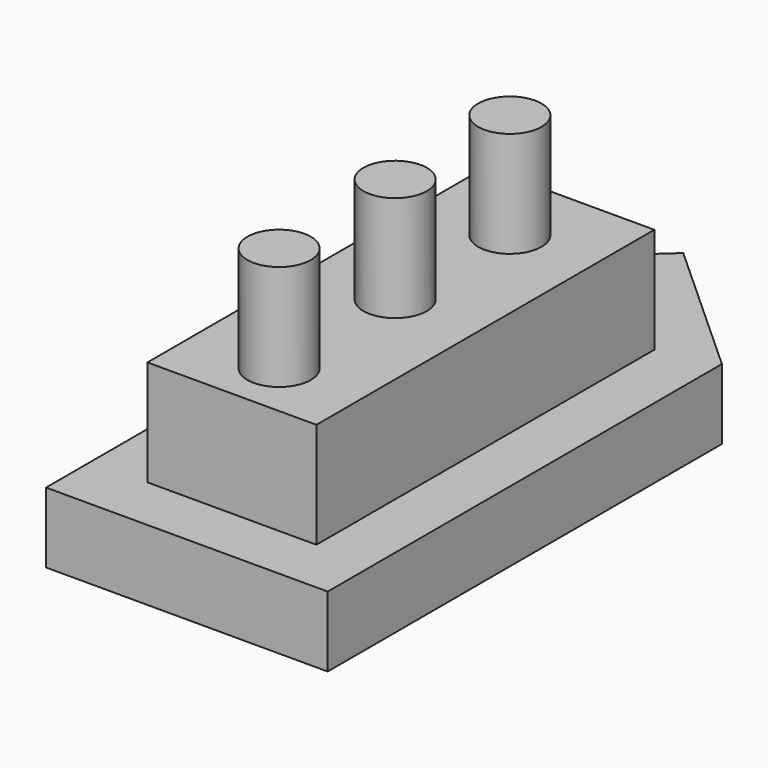
from build123d import *

# Parameters (mm, degrees)
F1_DEPTH     = 10
F2_W         = 24
F2_H         = 60
F3_DEPTH     = 25
F4_R         = 4.5
F5_DEPTH     = 15
F6_TEXT_SIZE = 11.8107172764
F7_DEPTH     = 5


# Not quite as in the source:
# - Text() gives the source's letters only with a copy of the font that has no kerning and outlines rounded to 1/6400 em; it was checked with that copy


with BuildPart() as f1:
    # F0 (on Top) → F1 (new body)
    with BuildSketch(Plane.XY):
        Polygon((-0.2903077006, 42.5211455371), (-20.2903077006, 24.3827883899), (-20.2903077006, -45.6172116101), (19.7096922994, -45.6172116101), (19.7096922994, 24.3827883899), align=None)
    extrude(amount=F1_DEPTH)

    # F2 (on Top) → F3 (join)
    with BuildSketch(Plane.XY):
        with Locations((-0.2903077006, -7.6172116101)):
            Rectangle(F2_W, F2_H)
    extrude(amount=F3_DEPTH)

    # F4 (on face) → F5 (join)
    with BuildSketch(Plane.XY.offset(25)):
        with Locations((0, 11.3601614535)):
            Circle(F4_R)
        with Locations((-0.2903077006, -8.6398385465)):
            Circle(F4_R)
        with Locations((0, -29.6020694077)):
            Circle(F4_R)
    extrude(amount=F5_DEPTH)

    # F6 (on face) → F7 (cut)
    with BuildSketch(Plane(origin=(-12.2903077006, 0, 0), x_dir=(0, -1, 0), z_dir=(-1, 0, 0))):
        with Locations((-22.3827883899, 12.8175793216)):
            Text('sara/lamia', F6_TEXT_SIZE, font='Open Sans', text_align=(TextAlign.LEFT, TextAlign.BOTTOM))
    extrude(amount=-F7_DEPTH, mode=Mode.SUBTRACT)


solid = f1.part
